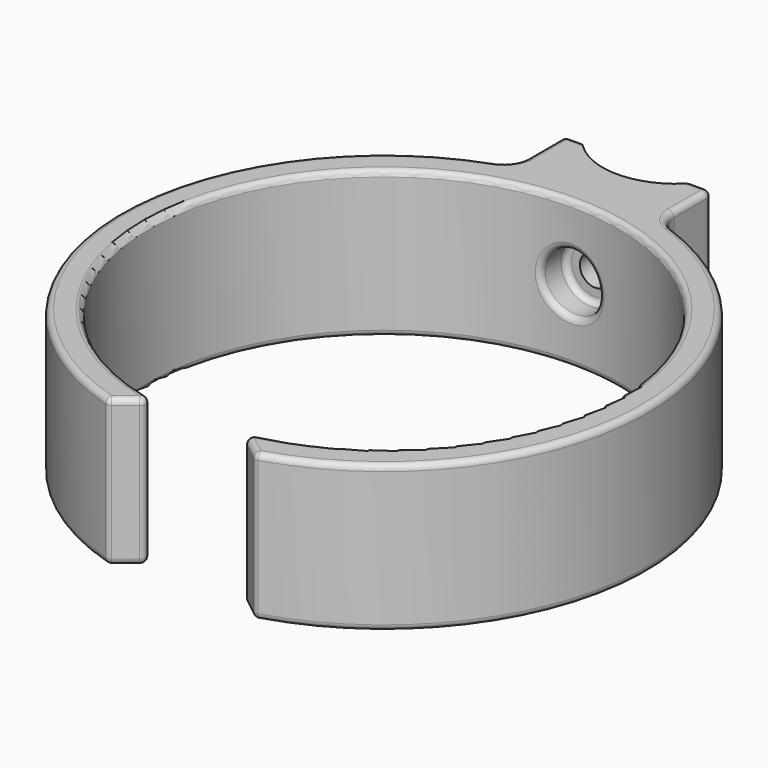
from build123d import *

# Parameters (mm, degrees)
F1_DEPTH        = 25
F2_R            = 4
F3_R            = 4
F4_R            = 1
F6_D            = 5.2
F6_START        = 54.8765563
F6_CBORE_D      = 10
F6_CBORE_DEPTH  = 5
F7_R            = 1
F8_D            = 25
F10_D           = 4
F10_DEPTH       = 12
F10_START       = 4.5000001
F10_CBORE_D     = 12
F10_CBORE_DEPTH = 1
F10_TIP         = 1.2017212381


with BuildPart() as f1:
    # F0 (on Top) → F1 (new body)
    with BuildSketch(Plane.XY):
        with BuildLine():
            ThreePointArc((-7.5, -24.4140279041), (0, 54.8765562097), (7.5, -24.4140279041))
            Line((7.5, -24.4140279041), (12.5, -28.3524849548))
            ThreePointArc((12.5, -28.3524849548), (45, 14.8765562097), (12.5, 58.1055973741))
            ThreePointArc((12.5, 58.1055973741), (0, 59.8765562097), (-12.5, 58.1055973741))
            ThreePointArc((-12.5, 58.1055973741), (-45, 14.8765562097), (-12.5, -28.3524849548))
            Line((-12.5, -28.3524849548), (-7.5, -24.4140279041))
        make_face()
        with BuildLine():
            ThreePointArc((-12.5, 58.1055973741), (0, 59.8765562097), (12.5, 58.1055973741))
            Line((12.5, 58.1055973741), (12.5, 69.1055973741))
            Line((12.5, 69.1055973741), (-12.5, 69.1055973741))
            Line((-12.5, 69.1055973741), (-12.5, 58.1055973741))
        make_face()
    extrude(amount=F1_DEPTH)

    # F2
    f2_edges = [f1.edges().sort_by_distance(p)[0] for p in [
        (-12.5, 58.105597, 12.5),
    ]]
    fillet(f2_edges, radius=F2_R)

    # F3
    f3_edges = [f1.edges().sort_by_distance(p)[0] for p in [
        (12.5, 58.105597, 12.5),
    ]]
    fillet(f3_edges, radius=F3_R)

    # F4
    f4_edges = [f1.edges().sort_by_distance(p)[0] for p in [
        (7.5, -24.414028, 12.5),
        (12.5, -28.352485, 12.5),
        (-7.5, -24.414028, 12.5),
        (-12.5, -28.352485, 12.5),
        (12.5, 69.105597, 12.5),
        (-12.5, 69.105597, 12.5),
    ]]
    fillet(f4_edges, radius=F4_R)

    # F6 (through all)
    # its depths count from where the whole tool has entered the part; down to there all is cleared
    with Locations(Plane.XZ.offset(-F6_START)):
        with Locations((0, 12.5)):
            CounterBoreHole(F6_D / 2, F6_CBORE_D / 2, F6_CBORE_DEPTH)

    # F7
    f7_edges = [f1.edges().sort_by_distance(p)[0] for p in [
        (0, 54.876556, 0),
        (-9.544225, -23.968106, 12.5),
        (9.544225, -23.968106, 12.5),
        (0, 54.876556, 25),
        (-5, 54.562826, 12.5),
        (12.5, 64.560266, 0),
        (12.207107, 68.812704, 0),
        (13.229851, 58.711433, 0),
        (44.985743, 13.743889, 0),
        (-12.207107, 68.812704, 0),
        (12.52662, -28.229516, 0),
        (-12.5, 64.560266, 0),
        (10.628922, -26.878653, 0),
        (-13.229851, 58.711433, 0),
        (8.805457, -24.727702, 0),
        (-44.985743, 13.743889, 0),
        (-12.52662, -28.229516, 0),
        (-8.805457, -24.727702, 0),
        (-10.628922, -26.878653, 0),
        (12.5, 64.560266, 25),
        (12.207107, 68.812704, 25),
        (13.229851, 58.711433, 25),
        (44.985743, 13.743889, 25),
        (-12.207107, 68.812704, 25),
        (12.52662, -28.229516, 25),
        (-12.5, 64.560266, 25),
        (10.628922, -26.878653, 25),
        (-13.229851, 58.711433, 25),
        (8.805457, -24.727702, 25),
        (-44.985743, 13.743889, 25),
        (-12.52662, -28.229516, 25),
        (-8.805457, -24.727702, 25),
        (-10.628922, -26.878653, 25),
        (-5, 59.876556, 12.5),
    ]]
    fillet(f7_edges, radius=F7_R)

    # F8 (through all)
    with Locations(Plane(origin=(0, 0, 0), x_dir=(1, 0, 0), z_dir=(0, 0, -1))):
        with Locations((0, -77.1055973741)):
            Hole(F8_D / 2)

    # F10
    # its depths count from where the whole tool has entered the part; down to there all is cleared
    with Locations(Plane(origin=(0, 69.1055973741, 0), x_dir=(-1, 0, 0), z_dir=(0, 1, 0)).offset(-F10_START)):
        with Locations((0, 12.5)):
            CounterBoreHole(F10_D / 2, F10_CBORE_D / 2, F10_CBORE_DEPTH, depth=F10_DEPTH)
            with Locations((0, 0, -(F10_DEPTH + F10_TIP / 2))):  # 118° drill point
                Cone(0, F10_D / 2, F10_TIP, mode=Mode.SUBTRACT)


solid = f1.part
